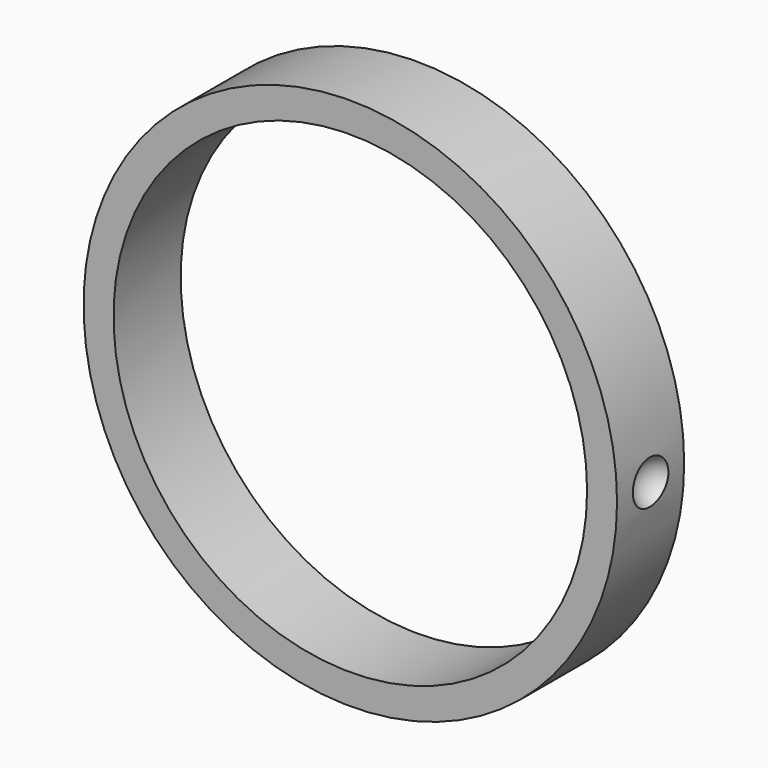
from build123d import *

# Parameters (mm, degrees)
F0_R     = 22.25
F0_R_2   = 19.75
F1_DEPTH = 7


# Not quite as in the source:
# - a feature of the source that left no trace in its solid (it failed there, or was rolled back) is left out
# - the program builds the solid bodies; features that only make, move or delete a surface that nothing else refers to are left out


with BuildPart() as f1:
    # F0 (on Front) → F1 (new body)
    with BuildSketch(Plane.XZ):
        Circle(F0_R)
        Circle(F0_R_2, mode=Mode.SUBTRACT)
    extrude(amount=F1_DEPTH)

    # F7 (on offset) → F8 (revolve, cut)
    with BuildSketch(Plane.YZ.offset(23)):
        with BuildLine():
            Line((-5.5, 0), (-1.5, 0))
            ThreePointArc((-1.5, 0), (-3.5, 2), (-5.5, 0))
        make_face()
    revolve(axis=Axis((23, -3.487871727, 0), (0, -1, 0)), mode=Mode.SUBTRACT)

    # F9: F1 across plane


with BuildPart() as f1_1:
    add(f1.part)
    add(f1.part.mirror(Plane.YZ), mode=Mode.INTERSECT)


solid = f1_1.part
